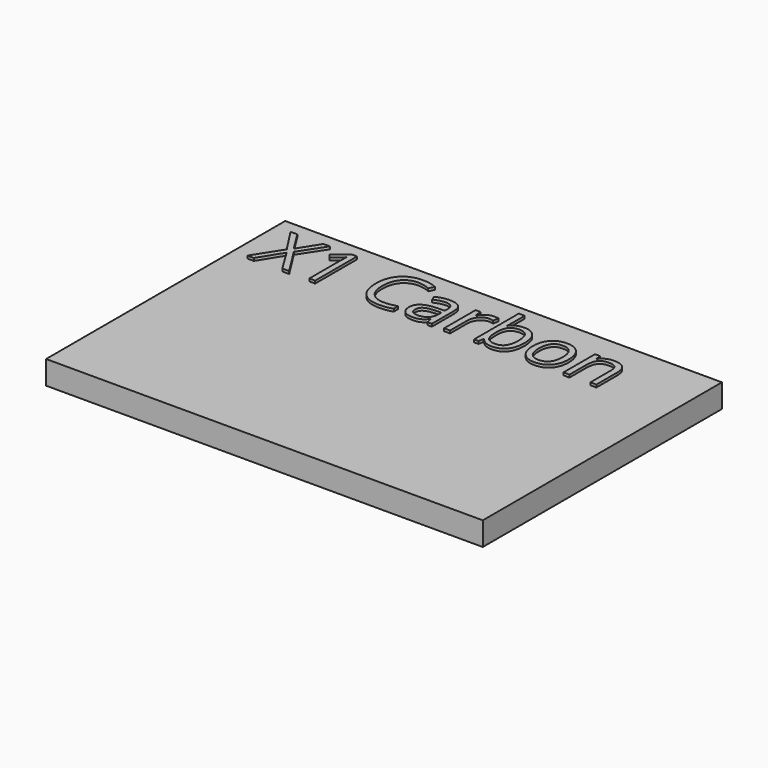
from build123d import *

# Parameters (mm, degrees)
F0_W         = 330.2
F0_H         = 226
F1_DEPTH     = 17.78
F2_TEXT_SIZE = 55.5555555556
F3_DEPTH     = 2


# Not quite as in the source:
# - Text() gives the source's letters only with a copy of the font that has no kerning and outlines rounded to 1/6400 em; it was checked with that copy


with BuildPart() as f1:
    # F0 (on Top) → F1 (new body)
    with BuildSketch(Plane.XY):
        with Locations((-8.9605848581, -2.4481430401)):
            Rectangle(F0_W, F0_H)
    extrude(amount=F1_DEPTH)

    # F2 (on face) → F3 (join)
    with BuildSketch(Plane.XY.offset(17.78)):
        with Locations((-161.6788887292, 59.0414568133)):
            Text('X1 Carbon', F2_TEXT_SIZE, font='Open Sans', text_align=(TextAlign.LEFT, TextAlign.BOTTOM))
    extrude(amount=F3_DEPTH)


solid = f1.part
